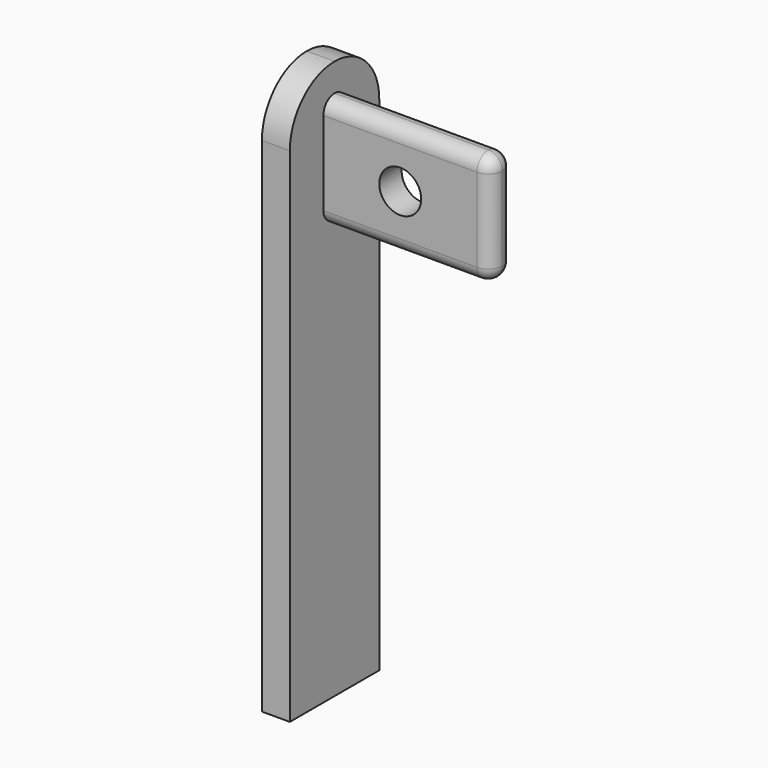
from build123d import *

# Parameters (mm, degrees)
F0_W     = 6.35
F0_H     = 127
F1_DEPTH = 25.4
F2_R     = 12.69999
F3_W     = 6.35
F3_H     = 25.3775035135
F4_DEPTH = 38.1
F5_R     = 3.17499
F6_R     = 4.7625
F7_DEPTH = 25.4


# Not quite as in the source:
# - a fillet or chamfer is up to 0.001 mm smaller than in the source, because OpenCascade refuses the exact size


with BuildPart() as f1:
    # F0 (on Front) → F1 (new body)
    with BuildSketch(Plane.XZ):
        with Locations((3.175, 63.5)):
            Rectangle(F0_W, F0_H)
    extrude(amount=F1_DEPTH)

    # F2 (radius 12.7 in the source; OpenCascade refuses exactly that, so slightly less here)
    f2_edges = [f1.edges().sort_by_distance(p)[0] for p in [
        (3.175, -25.4, 127),
        (3.175, 0, 127),
    ]]
    fillet(f2_edges, radius=F2_R)

    # F3 (on face) → F4 (join)
    with BuildSketch(Plane.YZ.offset(6.35)):
        with Locations((-12.7, 107.9612482432)):
            Rectangle(F3_W, F3_H)
    extrude(amount=F4_DEPTH)

    # F5 (radius 3.175 in the source; OpenCascade refuses exactly that, so slightly less here)
    f5_edges = [f1.edges().sort_by_distance(p)[0] for p in [
        (25.4, -15.875, 120.65),
        (25.4, -9.525, 120.65),
        (25.4, -15.875, 95.272496),
        (25.4, -9.525, 95.272496),
        (44.45, -15.875, 107.961248),
        (44.45, -9.525, 107.961248),
        (44.45, -12.7, 95.272496),
        (44.45, -12.7, 120.65),
    ]]
    fillet(f5_edges, radius=F5_R)

    # F6 (on face) → F7 (cut)
    with BuildSketch(Plane.XZ.offset(15.875)):
        with Locations((23.8125, 107.9612482432)):
            Circle(F6_R)
    extrude(amount=-F7_DEPTH, mode=Mode.SUBTRACT)


solid = f1.part
